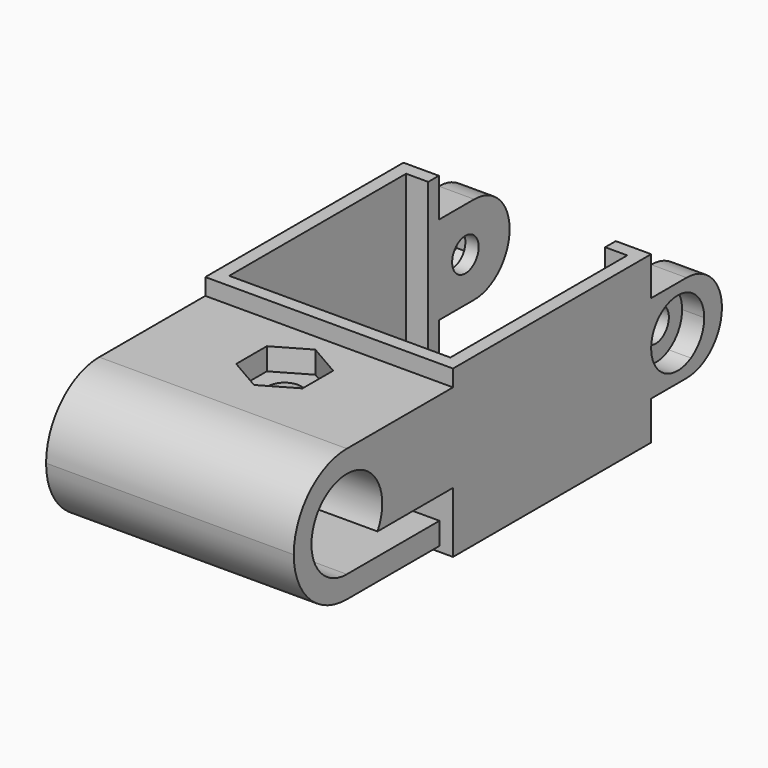
from build123d import *

# Parameters (mm, degrees)
F1_DEPTH  = 15
F3_DEPTH  = 22.4
F5_DEPTH  = 25
F6_START  = -10
F6_DEPTH  = 15
F7_W      = 3.2
F7_H      = 8
F8_DEPTH  = 8
F9_R      = 3.99999
F10_R     = 1.5
F11_DEPTH = 25
F12_DEPTH = 2
F13_START = -20.4
F13_DEPTH = 4.6


# Not quite as in the source:
# - a fillet or chamfer is up to 0.001 mm smaller than in the source, because OpenCascade refuses the exact size


with BuildPart() as f1:
    # F0 (on Top) → F1 (new body)
    with BuildSketch(Plane.XY):
        Polygon((20, 0), (0, 0), (0, 20), (2, 20), (2, 21.2), (-1.2, 21.2), (-1.2, -1.2), (21.2, -1.2), (21.2, 21.2), (18, 21.2), (18, 20), (20, 20), align=None)
    extrude(amount=F1_DEPTH)

    # F2 (on face) → F3 (join)
    with BuildSketch(Plane(origin=(-1.2, 0, 0), x_dir=(0, -1, 0), z_dir=(-1, 0, 0))):
        with BuildLine():
            Line((1.2, 5.5), (7.5431457505, 5.5))
            ThreePointArc((7.5431457505, 5.5), (8.3010205144, 10.9641016151), (13.2, 13.5))
            Line((13.2, 13.5), (1.2, 13.5))
            Line((1.2, 13.5), (1.2, 5.5))
        make_face()
        with BuildLine():
            ThreePointArc((17.2, 7.5), (16.0284271247, 4.6715728753), (13.2, 3.5))
            Line((13.2, 3.5), (8.727864045, 3.5))
            ThreePointArc((8.727864045, 3.5), (10.7505102572, 2.0227744249), (13.2, 1.5))
            ThreePointArc((13.2, 1.5), (17.4426406871, 3.2573593129), (19.2, 7.5))
            ThreePointArc((19.2, 7.5), (17.4426406871, 11.7426406871), (13.2, 13.5))
            ThreePointArc((13.2, 13.5), (8.3010205144, 10.9641016151), (7.5431457505, 5.5))
            Line((7.5431457505, 5.5), (9.7358983849, 5.5))
            ThreePointArc((9.7358983849, 5.5), (12.1647238196, 11.3637033052), (17.2, 7.5))
        make_face()
        with BuildLine():
            ThreePointArc((13.2, 1.5), (10.7505102572, 2.0227744249), (8.727864045, 3.5))
            Line((8.727864045, 3.5), (2.727864045, 3.5))
            Line((2.727864045, 3.5), (2.727864045, 1.5))
            Line((2.727864045, 1.5), (13.2, 1.5))
        make_face()
    extrude(amount=-F3_DEPTH)

    # F4 (on face) → F5 (cut)
    with BuildSketch(Plane(origin=(0, 0, 1.5), x_dir=(1, 0, 0), z_dir=(0, 0, -1))):
        with BuildLine():
            ThreePointArc((8.5, 6.227864045), (8.9393398282, 5.1672038732), (10, 4.727864045))
            Line((10, 4.727864045), (10, 6.227864045))
            Line((10, 6.227864045), (8.5, 6.227864045))
        make_face()
        with BuildLine():
            Line((10, 6.227864045), (10, 4.727864045))
            ThreePointArc((10, 4.727864045), (11.0606601718, 5.1672038732), (11.5, 6.227864045))
            ThreePointArc((11.5, 6.227864045), (10, 7.727864045), (8.5, 6.227864045))
            Line((8.5, 6.227864045), (10, 6.227864045))
        make_face()
    extrude(amount=-F5_DEPTH, mode=Mode.SUBTRACT)

    # F4 (on face) → F6 (cut)
    with BuildSketch(Plane(origin=(0, 0, 1.5), x_dir=(1, 0, 0), z_dir=(0, 0, -1)).offset(F6_START)):
        with BuildLine():
            Line((10, 4.727864045), (10, 2.7637624299))
            Line((10, 2.7637624299), (13, 4.4958132374))
            Line((13, 4.4958132374), (13, 7.9599148526))
            Line((13, 7.9599148526), (10, 9.6919656601))
            Line((10, 9.6919656601), (7, 7.9599148526))
            Line((7, 7.9599148526), (7, 6.227864045))
            Line((7, 6.227864045), (8.5, 6.227864045))
            ThreePointArc((8.5, 6.227864045), (10, 7.727864045), (11.5, 6.227864045))
            ThreePointArc((11.5, 6.227864045), (11.0606601718, 5.1672038732), (10, 4.727864045))
        make_face()
        with BuildLine():
            Line((7, 4.4958132374), (10, 2.7637624299))
            Line((10, 2.7637624299), (10, 4.727864045))
            ThreePointArc((10, 4.727864045), (8.9393398282, 5.1672038732), (8.5, 6.227864045))
            Line((8.5, 6.227864045), (7, 6.227864045))
            Line((7, 6.227864045), (7, 4.4958132374))
        make_face()
    extrude(amount=-F6_DEPTH, mode=Mode.SUBTRACT)

    # F7 (on face) → F8 (join)
    with BuildSketch(Plane(origin=(0, 21.2, 0), x_dir=(-1, 0, 0), z_dir=(0, 1, 0))):
        with Locations((-19.6, 7.5)):
            Rectangle(F7_W, F7_H)
        with Locations((-0.4, 7.5)):
            Rectangle(F7_W, F7_H)
    extrude(amount=F8_DEPTH)

    # F9 (radius 4 in the source; OpenCascade refuses exactly that, so slightly less here)
    f9_edges = [f1.edges().sort_by_distance(p)[0] for p in [
        (19.6, 29.2, 11.5),
        (19.6, 29.2, 3.5),
        (0.4, 29.2, 11.5),
        (0.4, 29.2, 3.5),
    ]]
    fillet(f9_edges, radius=F9_R)

    # F10 (on face) → F11 (cut)
    with BuildSketch(Plane.YZ.offset(21.2)):
        with Locations((24.2, 7.5)):
            Circle(F10_R)
    extrude(amount=-F11_DEPTH, mode=Mode.SUBTRACT)

    # F10 (on face) → F12 (cut)
    with BuildSketch(Plane.YZ.offset(21.2)):
        with BuildLine():
            ThreePointArc((25.7000000635, 4.9019238253), (26.7980762297, 6.0000000317), (27.2, 7.5))
            ThreePointArc((27.2, 7.5), (26.7980761988, 9.0000000218), (25.6999999564, 10.0980762365))
            ThreePointArc((25.6999999564, 10.0980762365), (24.2, 10.5), (22.7000000436, 10.0980762365))
            ThreePointArc((22.7000000436, 10.0980762365), (21.6019238012, 9.0000000218), (21.2, 7.5))
            ThreePointArc((21.2, 7.5), (21.6019238012, 5.9999999782), (22.7000000436, 4.9019237635))
            ThreePointArc((22.7000000436, 4.9019237635), (24.2000000618, 4.5), (25.7000000635, 4.9019238253))
        make_face()
        with Locations((24.2, 7.5)):
            Circle(F10_R, mode=Mode.SUBTRACT)
    extrude(amount=-F12_DEPTH, mode=Mode.SUBTRACT)

    # F10 (on face) → F13 (cut)
    with BuildSketch(Plane.YZ.offset(21.2).offset(F13_START)):
        with BuildLine():
            ThreePointArc((21.2, 7.5), (21.6019238012, 9.0000000218), (22.7000000436, 10.0980762365))
            Line((22.7000000436, 10.0980762365), (21.2, 9.2320508076))
            Line((21.2, 9.2320508076), (21.2, 7.5))
        make_face()
        with BuildLine():
            ThreePointArc((22.7000000436, 10.0980762365), (24.2, 10.5), (25.6999999564, 10.0980762365))
            Line((25.6999999564, 10.0980762365), (24.2, 10.9641016151))
            Line((24.2, 10.9641016151), (22.7000000436, 10.0980762365))
        make_face()
        with BuildLine():
            ThreePointArc((25.6999999564, 10.0980762365), (26.7980761988, 9.0000000218), (27.2, 7.5))
            Line((27.2, 7.5), (27.2, 9.2320508076))
            Line((27.2, 9.2320508076), (25.6999999564, 10.0980762365))
        make_face()
        with BuildLine():
            ThreePointArc((25.7000000635, 4.9019238253), (26.7980762297, 6.0000000317), (27.2, 7.5))
            ThreePointArc((27.2, 7.5), (26.7980761988, 9.0000000218), (25.6999999564, 10.0980762365))
            ThreePointArc((25.6999999564, 10.0980762365), (24.2, 10.5), (22.7000000436, 10.0980762365))
            ThreePointArc((22.7000000436, 10.0980762365), (21.6019238012, 9.0000000218), (21.2, 7.5))
            ThreePointArc((21.2, 7.5), (21.6019238012, 5.9999999782), (22.7000000436, 4.9019237635))
            ThreePointArc((22.7000000436, 4.9019237635), (24.2000000618, 4.5), (25.7000000635, 4.9019238253))
        make_face()
        with Locations((24.2, 7.5)):
            Circle(F10_R, mode=Mode.SUBTRACT)
        with BuildLine():
            Line((24.2, 4.0358983849), (25.7000000635, 4.9019238253))
            ThreePointArc((25.7000000635, 4.9019238253), (24.2000000618, 4.5), (22.7000000436, 4.9019237635))
            Line((22.7000000436, 4.9019237635), (24.2, 4.0358983849))
        make_face()
        with BuildLine():
            Line((21.2, 5.7679491924), (22.7000000436, 4.9019237635))
            ThreePointArc((22.7000000436, 4.9019237635), (21.6019238012, 5.9999999782), (21.2, 7.5))
            Line((21.2, 7.5), (21.2, 5.7679491924))
        make_face()
        with BuildLine():
            Line((27.2, 5.7679491924), (27.2, 7.5))
            ThreePointArc((27.2, 7.5), (26.7980762297, 6.0000000317), (25.7000000635, 4.9019238253))
            Line((25.7000000635, 4.9019238253), (27.2, 5.7679491924))
        make_face()
    extrude(amount=-F13_DEPTH, mode=Mode.SUBTRACT)


solid = f1.part
